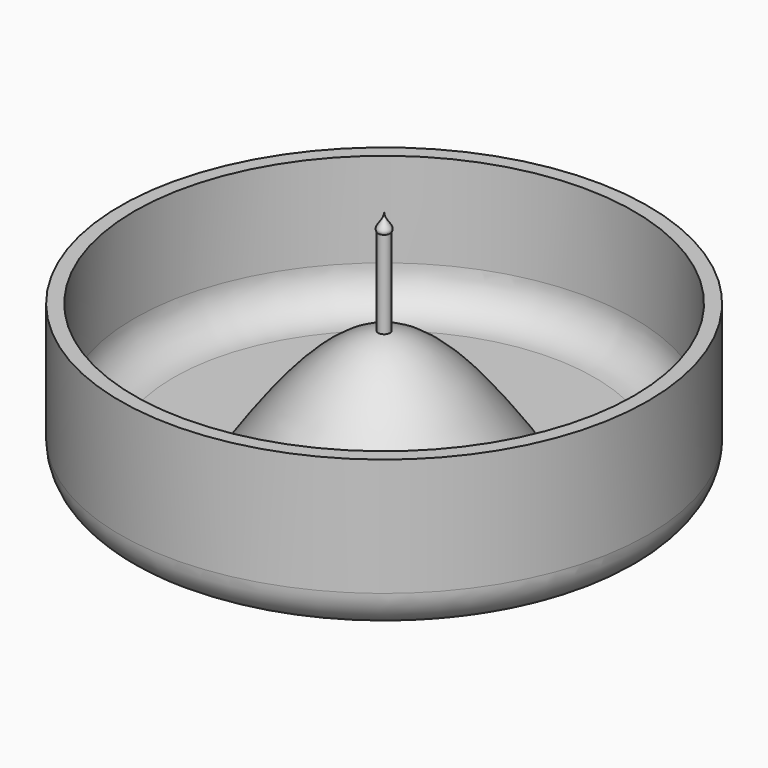
from build123d import *

# Parameters (mm, degrees)
F0_R     = 42.672
F0_R_2   = 40.386
F2_DEPTH = 25.4
F3_DEPTH = 3.81
F5_R     = 6.35


# Not quite as in the source:
# - a feature names something its author has since deleted; it is built from what else it names


with BuildPart() as f2:
    # F0 (on Top) → F2 (new body)
    with BuildSketch(Plane.XY):
        Circle(F0_R)
        Circle(F0_R_2, mode=Mode.SUBTRACT)
    extrude(amount=F2_DEPTH)

    # F0 (on Top) → F3 (join)
    with BuildSketch(Plane.XY):
        Circle(F0_R_2)
    extrude(amount=F3_DEPTH)

    # F1 (on Front) → F4 (revolve)
    with BuildSketch(Plane.XZ):
        with BuildLine():
            Line((-22.661603124, 0), (-0.3999708066, 0))
            Line((-0.3999708066, 0), (0, 0))
            Line((0, 0), (0, 21.5927247815))
            add(Edge.make_bspline(
                [(-0.9605343803, 21.5162747094), (-0.7741159133, 21.5404865376), (-0.4544785974, 21.5726982013), (-0.1335448781, 21.5887811226), (0, 21.5927247815)],
                knots=[0.4844452831, 0.4844452831, 0.4844452831, 0.4844452831, 0.4961290643, 0.5044321792, 0.5044321792, 0.5044321792, 0.5044321792], degree=3))
            add(Edge.make_bspline(
                [(-22.661603124, 0), (-15.6758083409, 10.256190155), (-8.6900138326, 20.5123783076), (-0.9605343803, 21.5162747094)],
                knots=[0, 0, 0, 0, 0.4844452831, 0.4844452831, 0.4844452831, 0.4844452831], degree=3))
        make_face()
        with BuildLine():
            Line((-0.9605343803, 35.6623469879), (0, 35.6623469879))
            Line((0, 35.6623469879), (0, 38.5057479143))
            add(Edge.make_bspline(
                [(0, 38.5057479143), (0, 37.0840474511), (-1.5196733875, 36.4921689034), (-0.9605343803, 35.6623469879)],
                knots=[0, 0, 0, 0, 3.0012589232, 3.0012589232, 3.0012589232, 3.0012589232], degree=3))
        make_face()
        with BuildLine():
            add(Edge.make_bspline(
                [(-0.9605343803, 21.5162747094), (-0.7741159133, 21.5404865376), (-0.4544785974, 21.5726982013), (-0.1335448781, 21.5887811226), (0, 21.5927247815)],
                knots=[0.4844452831, 0.4844452831, 0.4844452831, 0.4844452831, 0.4961290643, 0.5044321792, 0.5044321792, 0.5044321792, 0.5044321792], degree=3))
            Line((0, 21.5927247815), (0, 35.6623469879))
            Line((0, 35.6623469879), (-0.9605343803, 35.6623469879))
            Line((-0.9605343803, 35.6623469879), (-0.9605343803, 21.5162747094))
        make_face()
    revolve(axis=Axis((0, 0, 17.8311734939), (0, 0, -1)))

    # F5
    f5_edges = [f2.edges().sort_by_distance(p)[0] for p in [
        (-40.386, 0, 3.81),
        (-42.672, 0, 0),
    ]]
    fillet(f5_edges, radius=F5_R)


solid = f2.part
